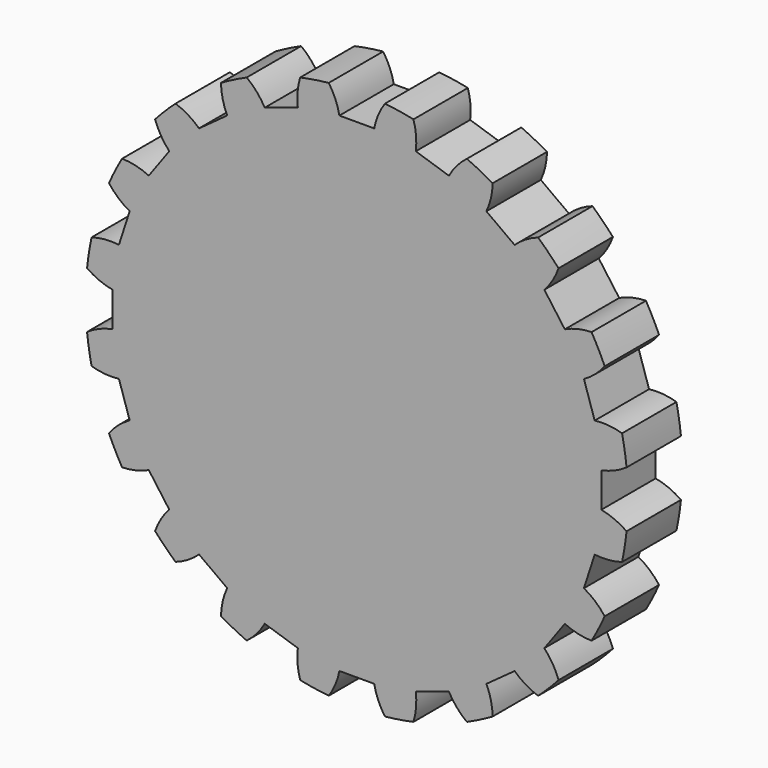
from build123d import *

# Parameters (mm, degrees)
F0_R            = 60.8062922789
F1_DEPTH        = 15.24
F3_DEPTH        = 15.241
F3_COPIES_COUNT = 20


# Not quite as in the source:
# - a pattern or mirror of a feature is missing from the dataset's text; its kind, count and spacing are read off the source's solid


with BuildPart() as f1:
    # F0 (on Front) → F1 (new body)
    with BuildSketch(Plane.XZ):
        Circle(F0_R)
    extrude(amount=F1_DEPTH)

    # F2 (on face) → F3 (cut, through all)
    with BuildSketch(Plane.XZ.offset(15.24)):
        with BuildLine():
            ThreePointArc((-10.0692585111, 64.2209947109), (-8.0132671596, 62.5211963323), (-6.2964195687, 60.4794203124))
            ThreePointArc((-6.2964195687, 60.4794203124), (0, 60.8062922789), (6.2964195687, 60.4794203124))
            ThreePointArc((6.2964195687, 60.4794203124), (8.0132671596, 62.5211963323), (10.0692585111, 64.2209947109))
            Line((10.0692585111, 64.2209947109), (-10.0692585111, 64.2209947109))
        make_face()
        with BuildLine():
            ThreePointArc((-6.2964195687, 60.4794203124), (-4.802623185, 57.7701032506), (-3.9057508111, 54.8091158271))
            Line((-3.9057508111, 54.8091158271), (0, 54.8091158271))
            Line((0, 54.8091158271), (3.9057508111, 54.8091158271))
            ThreePointArc((3.9057508111, 54.8091158271), (4.802623185, 57.7701032506), (6.2964195687, 60.4794203124))
            ThreePointArc((6.2964195687, 60.4794203124), (0, 60.8062922789), (-6.2964195687, 60.4794203124))
        make_face()
    f3 = extrude(amount=-F3_DEPTH, mode=Mode.SUBTRACT)

    # F3_copies: F3 ×20 about axis
    f3_copies_axis = Axis((0, 0, 0), (0, 1, 0))
    for i in range(1, F3_COPIES_COUNT):
        add(f3.rotate(f3_copies_axis, i * 360 / F3_COPIES_COUNT), mode=Mode.SUBTRACT)


solid = f1.part
